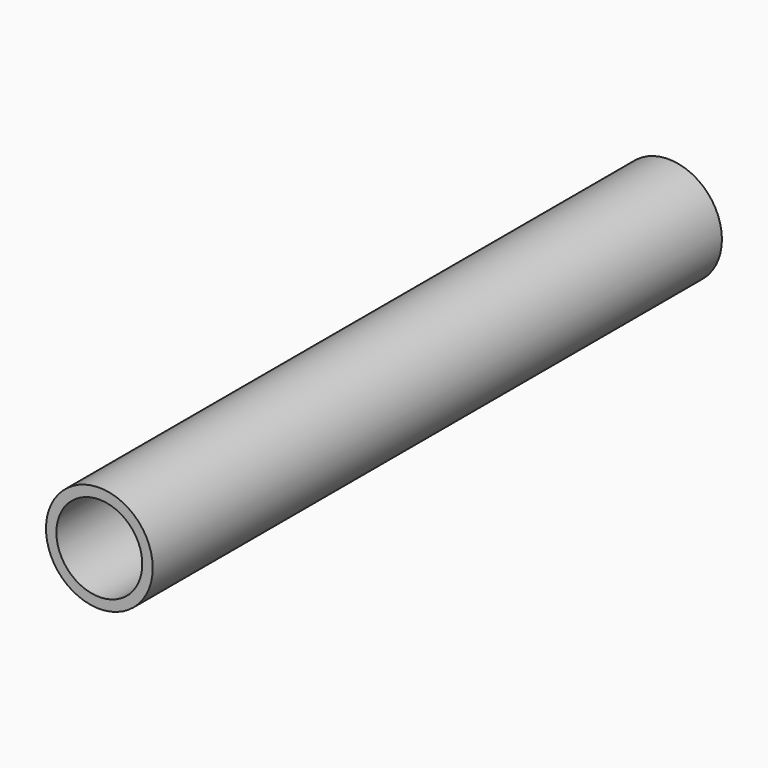
from build123d import *

# Parameters (mm, degrees)
F0_R     = 3.81
F1_DEPTH = 25.4
F3_DEPTH = 25.4
F4_R     = 3.0643911348
F5_DEPTH = 50.801


# Not quite as in the source:
# - the program builds the solid bodies; features that only make, move or delete a surface that nothing else refers to are left out


with BuildPart() as f1:
    # F0 (on Front) → F1 (new body)
    with BuildSketch(Plane.XZ):
        Circle(F0_R)
    extrude(amount=F1_DEPTH)

    # F3 (add): a face of the model
    f3_faces = [f1.faces().sort_by_distance(p)[0] for p in [
        (0, 0, 0),
    ]]
    extrude(f3_faces, amount=F3_DEPTH)

    # F4 (on face) → F5 (cut, through all)
    with BuildSketch(Plane(origin=(0, 25.4, 0), x_dir=(-1, 0, 0), z_dir=(0, 1, 0))):
        Circle(F4_R)
    extrude(amount=-F5_DEPTH, mode=Mode.SUBTRACT)


solid = f1.part
